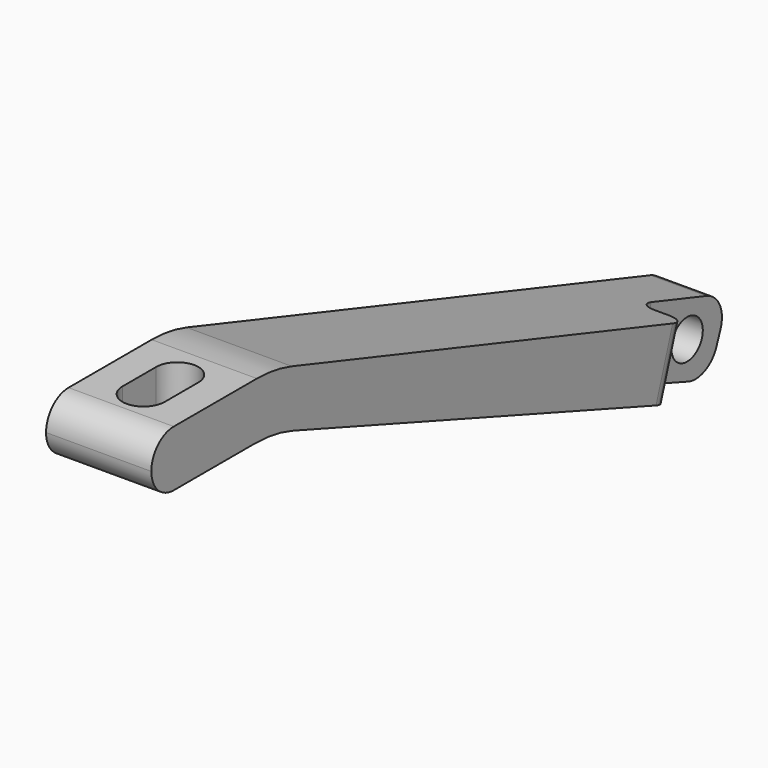
from build123d import *

# Parameters (mm, degrees)
F1_DEPTH = 15
F3_DEPTH = 25
F4_R     = 3.99999
F5_W     = 7.0163438655
F5_H     = 17.1485144225
F6_DEPTH = 25
F7_R     = 2.6
F8_R     = 2.8
F9_DEPTH = 25
F10_R    = 20
F11_R    = 4


# Not quite as in the source:
# - a fillet or chamfer is up to 0.001 mm smaller than in the source, because OpenCascade refuses the exact size


with BuildPart() as f1:
    # F0 (on Right) → F1 (new body)
    with BuildSketch(Plane.YZ):
        Polygon((-44.9859467229, 8), (-66.9859467229, 8), (-66.9859467229, 0), (-44.9859467229, 0), (41.0894067598, -30.7737162478), (42.3002508738, -27.5966470596), (43.3758810707, -24.7743584453), (44.6834651639, -21.3434583933), align=None)
    extrude(amount=F1_DEPTH)

    # F2 (on face) → F3 (cut)
    with BuildSketch(Plane(origin=(0, 0, 0), x_dir=(1, 0, 0), z_dir=(0, 0, -1))):
        with BuildLine():
            Line((4.5, 58.9859467229), (4.5, 52.9859467229))
            ThreePointArc((4.5, 52.9859467229), (7.5, 49.9859467229), (10.5, 52.9859467229))
            Line((10.5, 52.9859467229), (10.5, 58.9859467229))
            ThreePointArc((10.5, 58.9859467229), (7.5, 61.9859467229), (4.5, 58.9859467229))
        make_face()
    extrude(amount=-F3_DEPTH, mode=Mode.SUBTRACT)

    # F4 (radius 4 in the source; OpenCascade refuses exactly that, so slightly less here)
    f4_edges = [f1.edges().sort_by_distance(p)[0] for p in [
        (7.5, -66.985947, 0),
        (7.5, -66.985947, 8),
    ]]
    fillet(f4_edges, radius=F4_R)

    # F5 (on face) → F6 (cut)
    with BuildSketch(Plane(origin=(0, -1.9867064016, -6.0710906068), x_dir=(1, 0, 0), z_dir=(0, 0.3110113487, 0.9504061979))):
        with Locations((11.4918280672, 40.5312428041)):
            Rectangle(F5_W, F5_H)
        Polygon((15, 49.1055000154), (15, 31.9569855928), (21.9836561345, 31.9569855928), (21.9836561345, 65.9569855928), (7.9836561345, 65.9569855928), (7.9836561345, 49.1055000154), align=None)
    extrude(amount=-F6_DEPTH, mode=Mode.SUBTRACT)

    # F7
    f7_edges = [f1.edges().sort_by_distance(p)[0] for p in [
        (7.983656, 26.888111, -20.58561),
        (15, 26.888111, -20.58561),
    ]]
    fillet(f7_edges, radius=F7_R)

    # F8 (on face) → F9 (cut)
    with BuildSketch(Plane.YZ.offset(15)):
        with Locations((37.2460966017, -24.0897076146)):
            Circle(F8_R)
    extrude(amount=-F9_DEPTH, mode=Mode.SUBTRACT)

    # F10
    f10_edges = [f1.edges().sort_by_distance(p)[0] for p in [
        (7.5, -44.985947, 8),
        (7.5, -44.985947, 0),
    ]]
    fillet(f10_edges, radius=F10_R)

    # F11
    f11_edges = [f1.edges().sort_by_distance(p)[0] for p in [
        (3.991828, 41.089407, -30.773716),
        (3.991828, 44.683465, -21.343458),
    ]]
    fillet(f11_edges, radius=F11_R)


solid = f1.part
